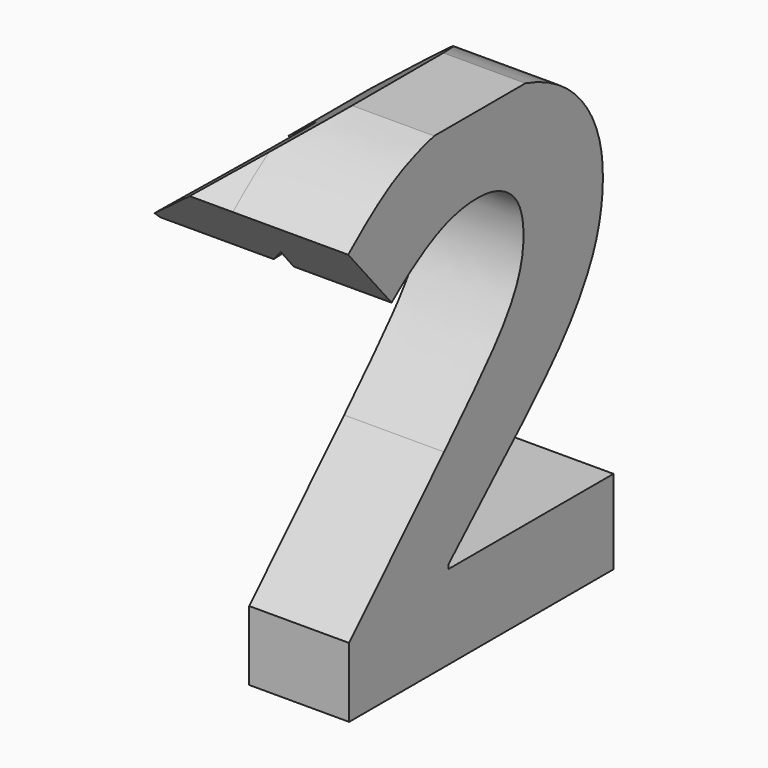
from build123d import *

# Parameters (mm, degrees)
F1_TEXT_SIZE  = 138.8888888889
F2_DEPTH      = 50
F2_DEPTH_BACK = 50
F3_START      = -50
F0_TEXT_SIZE  = 138.8888888889
F3_DEPTH      = 100


# Not quite as in the source:
# - Text() gives the source's letters only with a copy of the font that has no kerning and outlines rounded to 1/6400 em; it was checked with that copy


with BuildPart() as f2:
    # F1 (on Right) → F2 (new body, two sides)
    with BuildSketch(Plane.YZ) as f2_sk:
        with Locations((-41.9379340278, -50)):
            Text('2', F1_TEXT_SIZE, font='Open Sans', font_style=FontStyle.BOLD, text_align=(TextAlign.LEFT, TextAlign.BOTTOM))
    extrude(amount=F2_DEPTH)
    extrude(f2_sk.sketch, amount=-F2_DEPTH_BACK)

    # F0 (on Front) → F3 (intersect)
    with BuildSketch(Plane.XZ.offset(F3_START)):
        with Locations((-33.1922743056, -50)):
            Text('1', F0_TEXT_SIZE, font='Open Sans', font_style=FontStyle.BOLD, text_align=(TextAlign.LEFT, TextAlign.BOTTOM))
    extrude(amount=F3_DEPTH, mode=Mode.INTERSECT)


solid = f2.part
